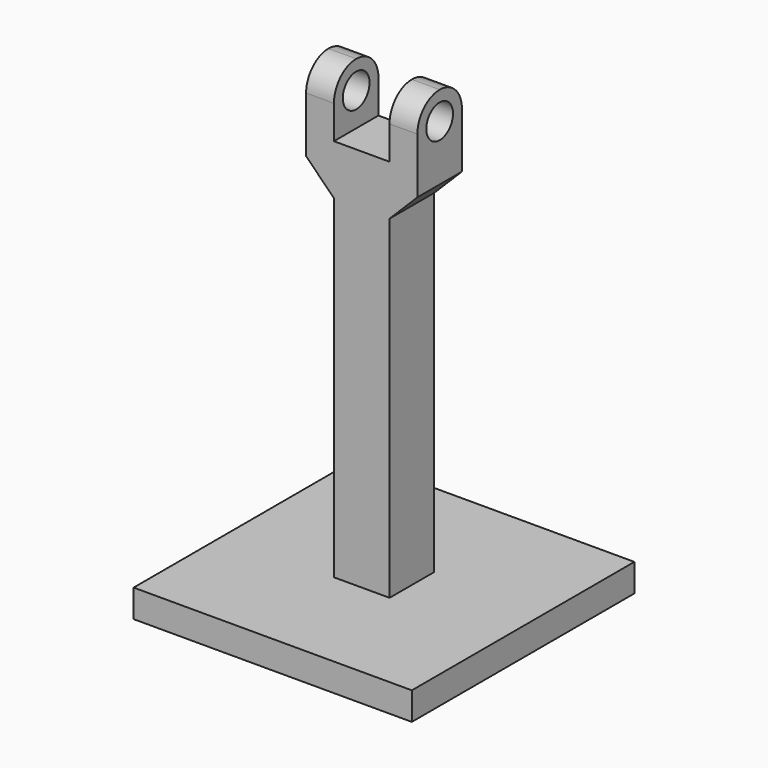
from build123d import *

# Parameters (mm, degrees)
F0_W      = 50
F0_H      = 50
F0_W_2    = 10
F0_H_2    = 10
F1_DEPTH  = 5
F2_DEPTH  = 75
F3_W      = 10
F3_H      = 5
F4_DEPTH  = 5
F5_W      = 10
F5_H      = 5
F6_DEPTH  = 5
F7_W      = 5
F7_H      = 10
F8_DEPTH  = 10
F10_D     = 6
F10_DEPTH = 20.001
F12_D     = 6
F13_R     = 4.99999
F14_DEPTH = 1
F15_DEPTH = 5
F16_SIZE  = 4.99999


# Not quite as in the source:
# - a fillet or chamfer is up to 0.001 mm smaller than in the source, because OpenCascade refuses the exact size


with BuildPart() as f1:
    # F0 (on Top) → F1 (new body)
    with BuildSketch(Plane.XY):
        Rectangle(F0_W, F0_H)
        Rectangle(F0_W_2, F0_H_2, mode=Mode.SUBTRACT)
    extrude(amount=F1_DEPTH)

    # F0 (on Top) → F2 (join)
    with BuildSketch(Plane.XY):
        Rectangle(F0_W_2, F0_H_2)
    extrude(amount=F2_DEPTH)

    # F3 (on face) → F4 (join)
    with BuildSketch(Plane.YZ.offset(5)):
        with Locations((0, 72.5)):
            Rectangle(F3_W, F3_H)
    extrude(amount=F4_DEPTH)

    # F5 (on face) → F6 (join)
    with BuildSketch(Plane(origin=(-5, 0, 0), x_dir=(0, -1, 0), z_dir=(-1, 0, 0))):
        with Locations((0, 72.5)):
            Rectangle(F5_W, F5_H)
    extrude(amount=F6_DEPTH)

    # F7 (on face) → F8 (join)
    with BuildSketch(Plane.XY.offset(75)):
        with Locations((7.5, 0)):
            Rectangle(F7_W, F7_H)
        with Locations((-7.5, 0)):
            Rectangle(F7_W, F7_H)
    extrude(amount=F8_DEPTH)

    # F10 (through all, one way)
    with BuildSketch(Plane(origin=(5, 0, 0), x_dir=(0, -1, 0), z_dir=(-1, 0, 0))):
        with Locations((0, 80)):
            Circle(F10_D / 2)
    extrude(amount=-F10_DEPTH, mode=Mode.SUBTRACT)

    # F12 (through all)
    with Locations(Plane.YZ.offset(-5)):
        with Locations((0, 80)):
            Hole(F12_D / 2)

    # F13 (radius 5 in the source; OpenCascade refuses exactly that, so slightly less here)
    f13_edges = [f1.edges().sort_by_distance(p)[0] for p in [
        (-7.5, -5, 85),
        (7.5, -5, 85),
        (7.5, 5, 85),
        (-7.5, 5, 85),
    ]]
    fillet(f13_edges, radius=F13_R)

    # F14 (cut): a face of the model
    f14_faces = [f1.faces().sort_by_distance(p)[0] for p in [
        (0, 0, 75),
    ]]
    extrude(f14_faces, amount=-F14_DEPTH, mode=Mode.SUBTRACT)

    # F15 (add): faces of the model
    f15_faces = [f1.faces().sort_by_distance(p)[0] for p in [
        (7.5, 0, 70),
        (-7.5, 0, 70),
    ]]
    extrude(f15_faces, amount=F15_DEPTH)

    # F16 (size 5 in the source; OpenCascade refuses exactly that, so slightly less here)
    f16_edges = [f1.edges().sort_by_distance(p)[0] for p in [
        (10, 0, 65),
        (-10, 0, 65),
    ]]
    chamfer(f16_edges, length=F16_SIZE)


solid = f1.part
